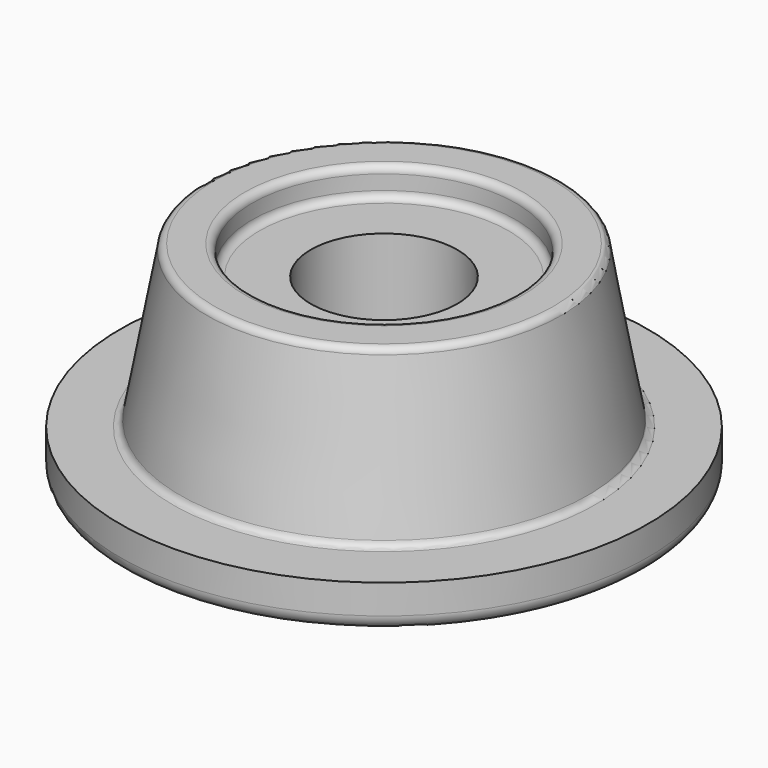
from build123d import *

# Parameters (mm, degrees)
F0_W = 3
F0_H = 1
F2_R = 1
F3_R = 0.5


# Not quite as in the source:
# - a fillet or chamfer that OpenCascade refuses, or shapes differently, is made with other operations: its cross-section is extruded or revolved along the edge and cut away or added


with BuildPart() as f1:
    # F0 (on Right) → F1 (revolve)
    with BuildSketch(Plane.YZ):
        Polygon((16, 0), (18, 0), (18, 3), (14, 3), (12, 14), (9, 14), (9, 12), (5, 12), (5, 0), (8, 0), (8, 1), (16, 1), align=None)
        with Locations((6.5, -0.5)):
            Rectangle(F0_W, F0_H)
    revolve(axis=Axis((0, 0, 16.8723911047), (0, 0, 1)))

    # F2
    f2_edges = [f1.edges().sort_by_distance(p)[0] for p in [
        (0, -18, 0),
    ]]
    fillet(f2_edges, radius=F2_R)

    # F3
    f3_edges = [f1.edges().sort_by_distance(p)[0] for p in [
        (0, -12, 14),
        (0, -14, 3),
        (0, -9, 12),
        (0, -9, 14),
    ]]
    fillet(f3_edges, radius=F3_R)

    # F4: fillet of radius 6 on 2 edges, made by hand

    # F4_s1 → F4_t2 (revolve)
    with BuildSketch(Plane.YZ):
        with BuildLine():
            ThreePointArc((12.472135955, 1), (10.0226462122, 0.4772255751), (8, -1))
            Line((8, -1), (8, 1))
            Line((8, 1), (12.472135955, 1))
        make_face()
    revolve(axis=Axis((0, 0, 1), (0, 0, 1)))

    # F4_s3 → F4_t4 (revolve)
    with BuildSketch(Plane.YZ):
        with BuildLine():
            ThreePointArc((16, 0), (14.4154260172, 0.7445626465), (12.6833752096, 1))
            Line((12.6833752096, 1), (16, 1))
            Line((16, 1), (16, 0))
        make_face()
    revolve(axis=Axis((0, 0, 1), (0, 0, 1)))


solid = f1.part
